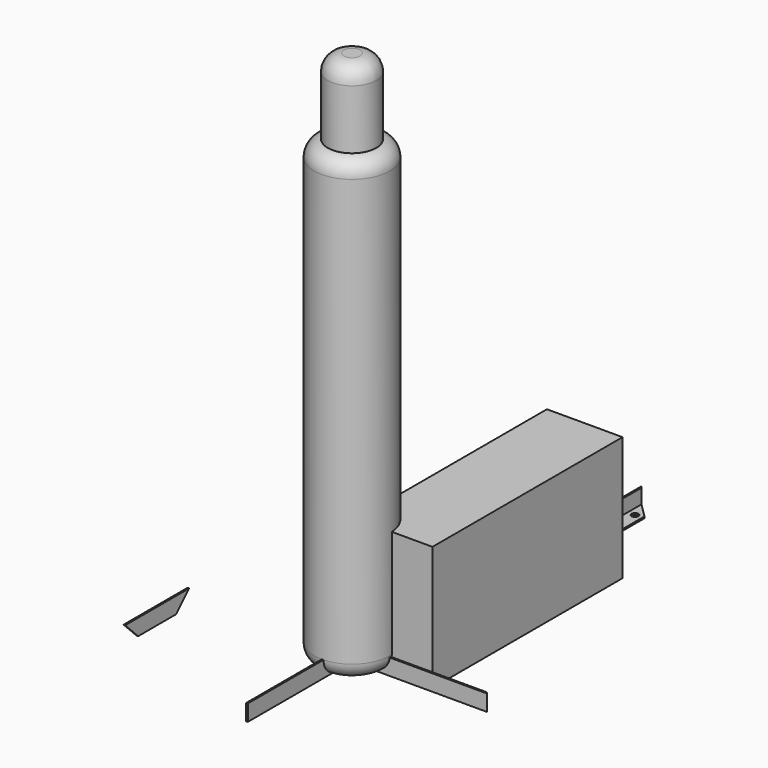
from build123d import *

# Parameters (mm, degrees)
F0_W      = 140
F0_H      = 440
F1_DEPTH  = 230
F3_DEPTH  = 460
F4_SIZE   = 29.99999
F6_DEPTH  = 250
F7_SIZE   = 29.99999
F9_DEPTH  = 300
F11_DEPTH = 600
F12_SIZE  = 29.99999
F13_W     = 3
F13_H     = 30
F14_DEPTH = 245
F15_W     = 3
F15_H     = 30
F16_DEPTH = 148
F17_SIZE  = 29.99999
F19_D     = 12.5
F19_2_D   = 12.5
F20_R     = 70
F21_DEPTH = 850
F22_R     = 45
F23_DEPTH = 140


# Not quite as in the source:
# - a fillet or chamfer that OpenCascade refuses, or shapes differently, is made with other operations: its cross-section is extruded or revolved along the edge and cut away or added
# - a fillet or chamfer is up to 0.001 mm smaller than in the source, because OpenCascade refuses the exact size


with BuildPart() as f1:
    # F0 (on Top) → F1 (new body)
    with BuildSketch(Plane.XY):
        with Locations((75, 225)):
            Rectangle(F0_W, F0_H)
    extrude(amount=F1_DEPTH)


with BuildPart() as f3:
    # F2 (on Front) → F3 (new body)
    with BuildSketch(Plane.XZ):
        Polygon((3, 0), (3, 27), (0, 27), (0, -3), (30, -3), (30, 0), align=None)
    extrude(amount=-F3_DEPTH)

    # F4 (size 30 in the source; OpenCascade refuses exactly that, so slightly less here)
    f4_edges = [f3.edges().sort_by_distance(p)[0] for p in [
        (30, 460, -1.5),
        (30, 0, -1.5),
    ]]
    chamfer(f4_edges, length=F4_SIZE)


with BuildPart() as f6:
    # F5 (on Right) → F6 (new body)
    with BuildSketch(Plane.YZ):
        Polygon((3, 27), (0, 27), (0, -3), (30, -3), (30, 0), (3, 0), align=None)
    extrude(amount=F6_DEPTH)

    # F7 (size 30 in the source; OpenCascade refuses exactly that, so slightly less here)
    f7_edges = [f6.edges().sort_by_distance(p)[0] for p in [
        (0, 30, -1.5),
        (250, 30, -1.5),
    ]]
    chamfer(f7_edges, length=F7_SIZE)

    # F19 (through all)
    with Locations(Plane.XY.offset(30.5873168707)):
        with Locations((72.0828511119, 35), (72.0828511119, 565)):
            Hole(F19_D / 2)


with BuildPart() as f9:
    # F8 (on Top) → F9 (new body)
    with BuildSketch(Plane.XY):
        Polygon((0, 30), (0, 0), (30, 0), (30, 3), (3, 3), (3, 30), align=None)
    extrude(amount=F9_DEPTH)


with BuildPart() as f11:
    # F10 (on Front) → F11 (new body)
    with BuildSketch(Plane.XZ):
        Polygon((58.5828511119, 30.5873168707), (58.5828511119, 57.5873168707), (55.5828511119, 57.5873168707), (55.5828511119, 27.5873168707), (85.5828511119, 27.5873168707), (85.5828511119, 30.5873168707), align=None)
    extrude(amount=-F11_DEPTH)

    # F12 (size 30 in the source; OpenCascade refuses exactly that, so slightly less here)
    f12_edges = [f11.edges().sort_by_distance(p)[0] for p in [
        (85.582851, 0, 29.087317),
        (85.582851, 600, 29.087317),
    ]]
    chamfer(f12_edges, length=F12_SIZE)

    # F19#2 (through all)
    with Locations(Plane.XY.offset(30.5873168707)):
        with Locations((72.0828511119, 35), (72.0828511119, 565)):
            Hole(F19_2_D / 2)


with BuildPart() as f14:
    # F13 (on Front) → F14 (new body)
    with BuildSketch(Plane.XZ):
        with Locations((1.5, 15)):
            Rectangle(F13_W, F13_H)
    extrude(amount=F14_DEPTH)


with BuildPart() as f16:
    # F15 (on Front) → F16 (new body)
    with BuildSketch(Plane.XZ):
        with Locations((-303.2166957855, 4.0501020849)):
            Rectangle(F15_W, F15_H)
    extrude(amount=F16_DEPTH)

    # F17 (size 30 in the source; OpenCascade refuses exactly that, so slightly less here)
    f17_edges = [f16.edges().sort_by_distance(p)[0] for p in [
        (-303.216696, 0, -10.949898),
        (-303.216696, -148, -10.949898),
    ]]
    chamfer(f17_edges, length=F17_SIZE)


with BuildPart() as f21:
    # F20 (on Top) → F21 (new body)
    with BuildSketch(Plane.XY):
        Circle(F20_R)
    extrude(amount=F21_DEPTH)

    # F22 (on face) → F23 (join)
    with BuildSketch(Plane.XY.offset(850)):
        Circle(F22_R)
    extrude(amount=F23_DEPTH)

    # F24: fillet of radius 30 on 3 edges, made by hand

    # F24_s1 → F24_t2 (revolve, cut)
    with BuildSketch(Plane.XZ):
        with BuildLine():
            ThreePointArc((70, 30), (61.2132034356, 8.7867965644), (40, 0))
            Line((40, 0), (70, 0))
            Line((70, 0), (70, 30))
        make_face()
    revolve(axis=Axis((0, 0, 0), (0, 0, 1)), mode=Mode.SUBTRACT)

    # F24_s3 → F24_t4 (revolve, cut)
    with BuildSketch(Plane.XZ):
        with BuildLine():
            ThreePointArc((70, 820.4196010845), (62.9128784748, 839.7845178155), (45, 850))
            Line((45, 850), (70, 850))
            Line((70, 850), (70, 820.4196010845))
        make_face()
    revolve(axis=Axis((0, 0, 850), (0, 0, 1)), mode=Mode.SUBTRACT)

    # F24_s5 → F24_t6 (revolve, cut)
    with BuildSketch(Plane.XZ):
        with BuildLine():
            ThreePointArc((45, 960), (36.2132034356, 981.2132034356), (15, 990))
            Line((15, 990), (45, 990))
            Line((45, 990), (45, 960))
        make_face()
    revolve(axis=Axis((0, 0, 990), (0, 0, 1)), mode=Mode.SUBTRACT)


solid = Compound([f1.part, f3.part, f6.part, f9.part, f11.part, f14.part, f16.part, f21.part])
